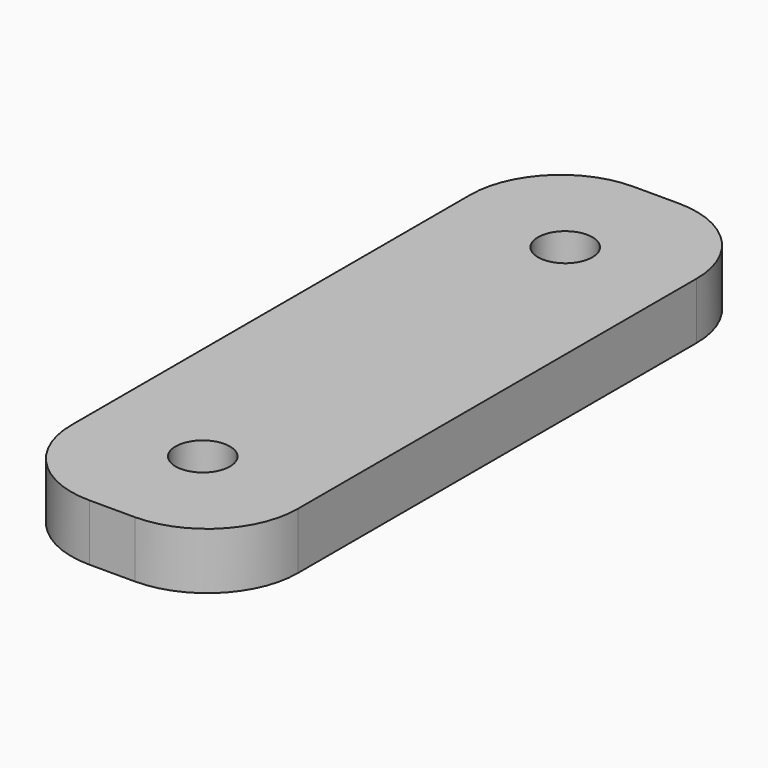
from build123d import *

# Parameters (mm, degrees)
F0_W     = 12.7
F0_H     = 38.1
F0_R     = 1.524
F1_DEPTH = 3.175
F2_R     = 5.08


# Not quite as in the source:
# - a length typed as a fraction of an inch, garbled in the dataset ("3 / 203.2 mm" for 3/8 in), is restored


with BuildPart() as f1:
    # F0 (on Top) → F1 (new body)
    with BuildSketch(Plane.XY):
        Rectangle(F0_W, F0_H)
        with Locations((0, -12.7)):
            Circle(F0_R, mode=Mode.SUBTRACT)
        with Locations((0, 12.7)):
            Circle(F0_R, mode=Mode.SUBTRACT)
    extrude(amount=F1_DEPTH)

    # F2
    f2_edges = [f1.edges().sort_by_distance(p)[0] for p in [
        (-6.35, 19.05, 1.5875),
        (6.35, 19.05, 1.5875),
        (-6.35, -19.05, 1.5875),
        (6.35, -19.05, 1.5875),
    ]]
    fillet(f2_edges, radius=F2_R)


solid = f1.part
